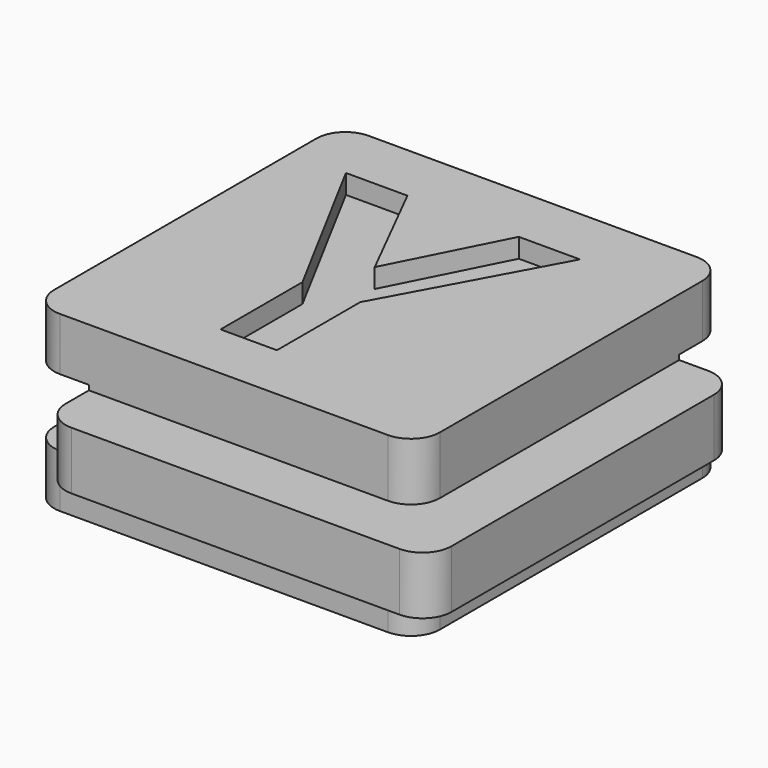
from build123d import *

# Parameters (mm, degrees)
F0_W         = 14
F0_H         = 3
F0_W_2       = 3
F1_DEPTH     = 20
F2_DEPTH     = 3
F3_W         = 3
F3_H         = 3
F4_DEPTH     = 100
F5_W         = 3
F5_H         = 3.5
F6_DEPTH     = 100
F7_R         = 1.5
F8_TEXT_SIZE = 19.4444444444
F9_DEPTH     = 1


# Not quite as in the source:
# - Text() gives the source's letters only with a copy of the font that has no kerning and outlines rounded to 1/6400 em; it was checked with that copy


with BuildPart() as f1:
    # F0 (on Front) → F1 (new body)
    with BuildSketch(Plane.XZ):
        Polygon((10, 1.5), (10, 4.5), (-10, 4.5), (-10, 1.5), (-7, 1.5), (7, 1.5), align=None)
        Rectangle(F0_W, F0_H)
        with Locations((11.5, 0)):
            Rectangle(F0_W_2, F0_H)
        with Locations((8.5, 0)):
            Rectangle(F0_W_2, F0_H)
        with Locations((-8.5, 0)):
            Rectangle(F0_W_2, F0_H)
        Polygon((10, -4.5), (10, -1.5), (7, -1.5), (-7, -1.5), (-10, -1.5), (-10, -4.5), align=None)
    extrude(amount=-F1_DEPTH)

    # F0 (on Front) → F2 (join)
    with BuildSketch(Plane.XZ):
        with Locations((-8.5, 0)):
            Rectangle(F0_W_2, F0_H)
        Rectangle(F0_W, F0_H)
        with Locations((8.5, 0)):
            Rectangle(F0_W_2, F0_H)
        with Locations((11.5, 0)):
            Rectangle(F0_W_2, F0_H)
    extrude(amount=F2_DEPTH)

    # F3 (on face) → F4 (cut)
    with BuildSketch(Plane.YZ.offset(13)):
        Polygon((23, -1.75), (23, 1.75), (17, 1.75), (17, 1.5), (20, 1.5), (20, -1.5), (17, -1.5), (17, -1.75), align=None)
        with Locations((18.5, 0)):
            Rectangle(F3_W, F3_H)
    extrude(amount=-F4_DEPTH, mode=Mode.SUBTRACT)

    # F5 (on face) → F6 (cut)
    with BuildSketch(Plane(origin=(0, 17, 0), x_dir=(-1, 0, 0), z_dir=(0, 1, 0))):
        with Locations((11.5, 0)):
            Rectangle(F5_W, F5_H)
        with Locations((8.5, 0)):
            Rectangle(F5_W, F5_H)
    extrude(amount=-F6_DEPTH, mode=Mode.SUBTRACT)

    # F7
    f7_edges = [f1.edges().sort_by_distance(p)[0] for p in [
        (-7, -3, 0),
        (13, -3, 0),
        (10, 0, 3),
        (10, 0, -3),
        (-10, 0, -3.125),
        (-10, 0, 3.125),
        (-7, 17, 0),
        (-10, 20, 3.125),
        (-10, 20, -3.125),
        (13, 17, 0),
        (10, 20, 3.125),
        (10, 20, -3.125),
    ]]
    fillet(f7_edges, radius=F7_R)

    # F8 (on face) → F9 (cut)
    with BuildSketch(Plane.XY.offset(4.5)):
        with Locations((-7.1801951318, 3)):
            Text('Y', F8_TEXT_SIZE, font='Open Sans', font_style=FontStyle.BOLD, text_align=(TextAlign.LEFT, TextAlign.BOTTOM))
    extrude(amount=-F9_DEPTH, mode=Mode.SUBTRACT)


solid = f1.part
